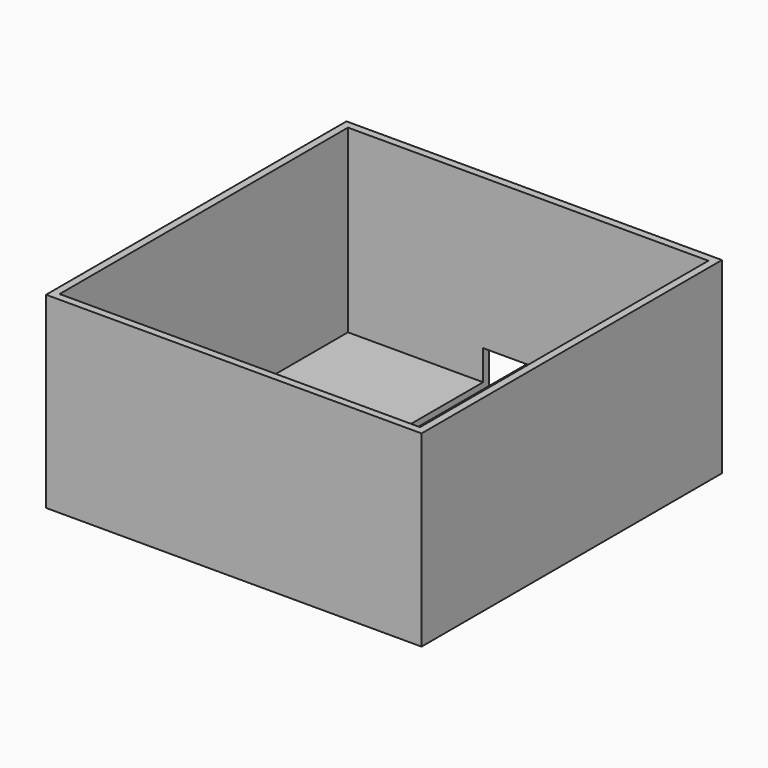
from build123d import *

# Parameters (mm, degrees)
F1_DEPTH      = 1
F3_DEPTH      = 25
F6_DEPTH      = 5
F6_DEPTH_BACK = 5
F8_W          = 12
F8_H          = 1
F9_DEPTH      = 20
F10_T1_DEPTH  = 13.0901699437
F10_T3_DEPTH  = 15
F10_T5_DEPTH  = 11.1803398875


# Not quite as in the source:
# - a fillet or chamfer that OpenCascade refuses, or shapes differently, is made with other operations: its cross-section is extruded or revolved along the edge and cut away or added


with BuildPart() as f1:
    # F0 (on Top) → F1 (new body)
    with BuildSketch(Plane.XY):
        Polygon((0, 50), (0, 0), (50, 0), (50, 50), (31, 50), (31, 35), (30, 35), (30, 60), (20, 60), (20, 35), (19, 35), (19, 50), align=None)
    extrude(amount=F1_DEPTH)

    # F2 (on Top) → F3 (join)
    with BuildSketch(Plane.XY):
        Polygon((0, 50), (0, 0), (50, 0), (50, 50), (31, 50), (31, 49), (49, 49), (49, 1), (1, 1), (1, 49), (19, 49), (19, 50), align=None)
    extrude(amount=F3_DEPTH)

    # F5 (on offset) → F6 (join, two sides)
    with BuildSketch(Plane.YZ.offset(25)) as f6_sk:
        Polygon((57.5, -5), (60, 0), (55, 0), (55, -5), align=None)
    extrude(amount=F6_DEPTH)
    extrude(f6_sk.sketch, amount=-F6_DEPTH_BACK)

    # F8 (on offset) → F9 (join)
    with BuildSketch(Plane.XY.offset(25)):
        with Locations((25, 49.5)):
            Rectangle(F8_W, F8_H)
    extrude(amount=-F9_DEPTH)

    # F10: fillet of radius 1 on 4 edges, made by hand

    # F10_s2 → F10_t1 (cut)
    with BuildSketch(Plane.YZ.offset(18.4549150281)):
        with BuildLine():
            ThreePointArc((57.7763932023, -4.4472135955), (57.4076971234, -4.8506508084), (56.8819660113, -5))
            Line((56.8819660113, -5), (57.5, -5))
            Line((57.5, -5), (57.7763932023, -4.4472135955))
        make_face()
    extrude(amount=F10_T1_DEPTH, mode=Mode.SUBTRACT)

    # F10_s4 → F10_t3 (cut)
    with BuildSketch(Plane.YZ.offset(17.5)):
        with BuildLine():
            ThreePointArc((56, -5), (55.2928932188, -4.7071067812), (55, -4))
            Line((55, -4), (55, -5))
            Line((55, -5), (56, -5))
        make_face()
        with BuildLine():
            ThreePointArc((59, 1), (59.7071067812, 0.7071067812), (60, 0))
            Line((60, 0), (60, 1))
            Line((60, 1), (59, 1))
        make_face()
    extrude(amount=F10_T3_DEPTH, mode=Mode.SUBTRACT)

    # F10_s6 → F10_t5 (cut)
    with BuildSketch(Plane.YZ.offset(19.4098300563)):
        with BuildLine():
            ThreePointArc((60, 0.2360679775), (59.9732489895, 0.006315057), (59.894427191, -0.211145618))
            Line((59.894427191, -0.211145618), (60, 0))
            Line((60, 0), (60, 0.2360679775))
        make_face()
    extrude(amount=F10_T5_DEPTH, mode=Mode.SUBTRACT)


solid = f1.part
